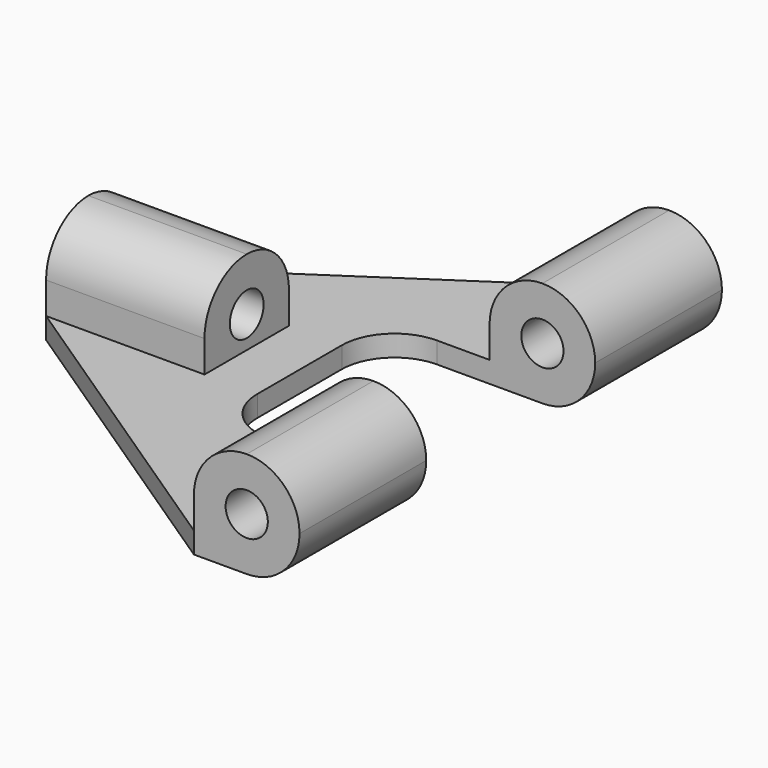
from build123d import *

# Parameters (mm, degrees)
F0_W      = 15
F0_H      = 3
F1_DEPTH  = 2
F2_W      = 15
F2_H      = 10
F3_DEPTH  = 8
F4_R      = 2
F5_DEPTH  = 25
F6_R      = 4.99999
F7_W      = 15
F7_H      = 8
F7_H_2    = 2
F8_DEPTH  = 10
F9_R      = 4.99999
F10_R     = 2
F11_DEPTH = 25
F12_W     = 15
F12_H     = 2
F12_H_2   = 8
F13_DEPTH = 10
F14_R     = 4.99999
F15_R     = 2
F16_DEPTH = 25
F17_R     = 5


# Not quite as in the source:
# - a fillet or chamfer is up to 0.001 mm smaller than in the source, because OpenCascade refuses the exact size


with BuildPart() as f1:
    # F0 (on Top) → F1 (new body)
    with BuildSketch(Plane.XY):
        Polygon((0, 25), (-30, 5), (-15, 5), (-15, 2), (-15, -2), (-15, -5), (-30, -5), (0, -25), (0, -10), (-10, -10), (-10, 10), (0, 10), align=None)
        with Locations((-22.5, 3.5)):
            Rectangle(F0_W, F0_H)
        Polygon((-30, 2), (-30, 0), (-30, -2), (-15, -2), (-15, 2), align=None)
        with Locations((-22.5, -3.5)):
            Rectangle(F0_W, F0_H)
    extrude(amount=F1_DEPTH)

    # F2 (on face) → F3 (join)
    with BuildSketch(Plane.XY.offset(2)):
        with Locations((-22.5, 0)):
            Rectangle(F2_W, F2_H)
    extrude(amount=F3_DEPTH)

    # F4 (on face) → F5 (cut)
    with BuildSketch(Plane(origin=(-30, 0, 0), x_dir=(0, -1, 0), z_dir=(-1, 0, 0))):
        with Locations((0, 5)):
            Circle(F4_R)
    extrude(amount=-F5_DEPTH, mode=Mode.SUBTRACT)

    # F6 (radius 5 in the source; OpenCascade refuses exactly that, so slightly less here)
    f6_edges = [f1.edges().sort_by_distance(p)[0] for p in [
        (-22.5, -5, 10),
        (-22.5, 5, 10),
    ]]
    fillet(f6_edges, radius=F6_R)

    # F7 (on face) → F8 (join)
    with BuildSketch(Plane.YZ):
        with Locations((-17.5, 6)):
            Rectangle(F7_W, F7_H)
        with Locations((-17.5, 1)):
            Rectangle(F7_W, F7_H_2)
    extrude(amount=F8_DEPTH)

    # F9 (radius 5 in the source; OpenCascade refuses exactly that, so slightly less here)
    f9_edges = [f1.edges().sort_by_distance(p)[0] for p in [
        (0, -17.5, 10),
        (10, -17.5, 10),
        (10, -17.5, 0),
    ]]
    fillet(f9_edges, radius=F9_R)

    # F10 (on face) → F11 (cut)
    with BuildSketch(Plane.XZ.offset(25)):
        with Locations((5, 5)):
            Circle(F10_R)
    extrude(amount=-F11_DEPTH, mode=Mode.SUBTRACT)

    # F12 (on face) → F13 (join)
    with BuildSketch(Plane.YZ):
        with Locations((17.5, 1)):
            Rectangle(F12_W, F12_H)
        with Locations((17.5, 6)):
            Rectangle(F12_W, F12_H_2)
    extrude(amount=F13_DEPTH)

    # F14 (radius 5 in the source; OpenCascade refuses exactly that, so slightly less here)
    f14_edges = [f1.edges().sort_by_distance(p)[0] for p in [
        (0, 17.5, 10),
        (10, 17.5, 10),
        (10, 17.5, 0),
    ]]
    fillet(f14_edges, radius=F14_R)

    # F15 (on face) → F16 (cut)
    with BuildSketch(Plane(origin=(0, 25, 0), x_dir=(-1, 0, 0), z_dir=(0, 1, 0))):
        with Locations((-5, 5)):
            Circle(F15_R)
    extrude(amount=-F16_DEPTH, mode=Mode.SUBTRACT)

    # F17
    f17_edges = [f1.edges().sort_by_distance(p)[0] for p in [
        (-10, 10, 1),
        (-10, -10, 1),
    ]]
    fillet(f17_edges, radius=F17_R)


solid = f1.part
